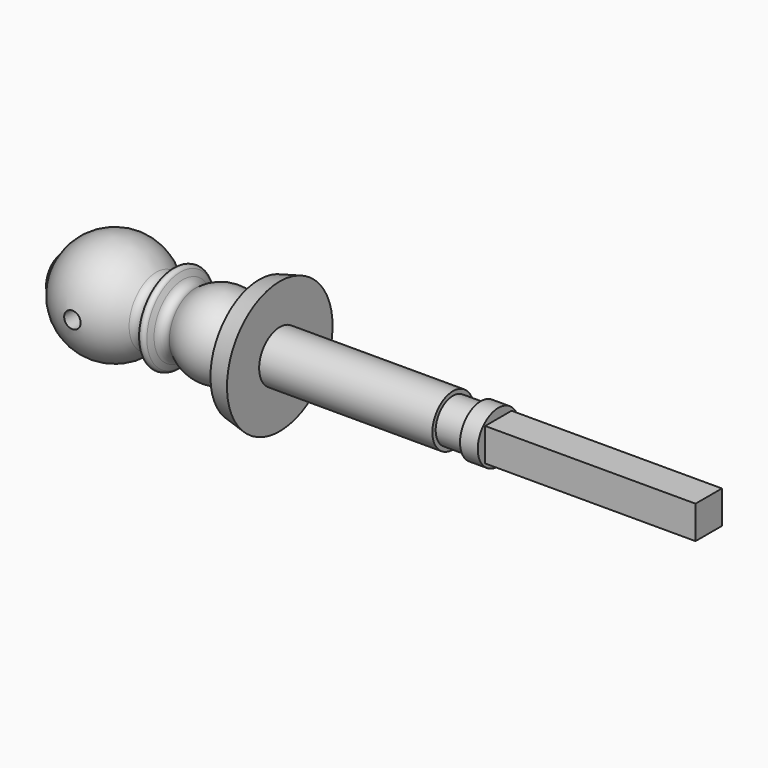
from build123d import *

# Parameters (mm, degrees)
F2_W          = 8
F2_H          = 8
F3_DEPTH      = 51
F4_W          = 45
F4_H          = 5
F8_R          = 2
F9_DEPTH      = 16.001
F9_DEPTH_BACK = 16.001


with BuildPart() as f1:
    # F0 (on Front) → F1 (revolve)
    with BuildSketch(Plane.XZ):
        Polygon((0, 6.25), (0, 0), (53, 0), (53, 6.25), (48.7, 6.25), (48.7, 5.25), (42, 5.25), (42, 6.25), align=None)
    revolve(axis=Axis((26.2976505187, 0, 0), (1, 0, 0)))

    # F2 (on face) → F3 (join)
    with BuildSketch(Plane.YZ.offset(53)):
        Rectangle(F2_W, F2_H)
    extrude(amount=F3_DEPTH)

    # F4 (on Front) → F5 (revolve)
    with BuildSketch(Plane.XZ):
        with Locations((-22.5, 2.5)):
            Rectangle(F4_W, F4_H)
    revolve(axis=Axis((-20.4847540462, 0, 0), (1, 0, 0)))


with BuildPart() as f7:
    # F6 (on Front) → F7 (revolve)
    with BuildSketch(Plane.XZ):
        with BuildLine():
            Line((-46, 5), (0, 5))
            Line((0, 5), (0, 16))
            Line((0, 16), (-5, 14.7562093884))
            Line((-5, 14.7562093884), (-5, 9.5))
            ThreePointArc((-5, 9.5), (-6.1179039309, 7.7050330017), (-8.2219065249, 7.9166666667))
            ThreePointArc((-8.2219065249, 7.9166666667), (-14.3314391493, 10), (-20.4409717737, 7.9166666667))
            ThreePointArc((-20.4409717737, 7.9166666667), (-22.1698295233, 7.5653164456), (-23.5042290197, 8.71934161))
            Line((-23.5042290197, 8.71934161), (-24.1066704056, 10.140329195))
            ThreePointArc((-24.1066704056, 10.140329195), (-25.0273457662, 10.75), (-25.9480211267, 10.140329195))
            Line((-25.9480211267, 10.140329195), (-26.5504625127, 8.71934161))
            ThreePointArc((-26.5504625127, 8.71934161), (-28.1079115815, 7.5202525788), (-29.9395714693, 8.2333333333))
            ThreePointArc((-29.9395714693, 8.2333333333), (-41.885230883, 12.8625776778), (-52, 5))
            Line((-52, 5), (-52.6602540378, 5))
            ThreePointArc((-52.6602540378, 5), (-53.6592582629, 2.588190451), (-54, 0))
            Line((-54, 0), (-48.2261434265, 0))
            Line((-48.2261434265, 0), (-46, 5))
        make_face()
    revolve(axis=Axis((-24.4397171773, 0, 0), (1, 0, 0)))

    # F8 (on Front) → F9 (cut, two sides)
    with BuildSketch(Plane.XZ) as f9_sk:
        with Locations((-40, 0)):
            Circle(F8_R)
    extrude(amount=-F9_DEPTH, mode=Mode.SUBTRACT)
    extrude(f9_sk.sketch, amount=F9_DEPTH_BACK, mode=Mode.SUBTRACT)


solid = Compound([f1.part, f7.part])
